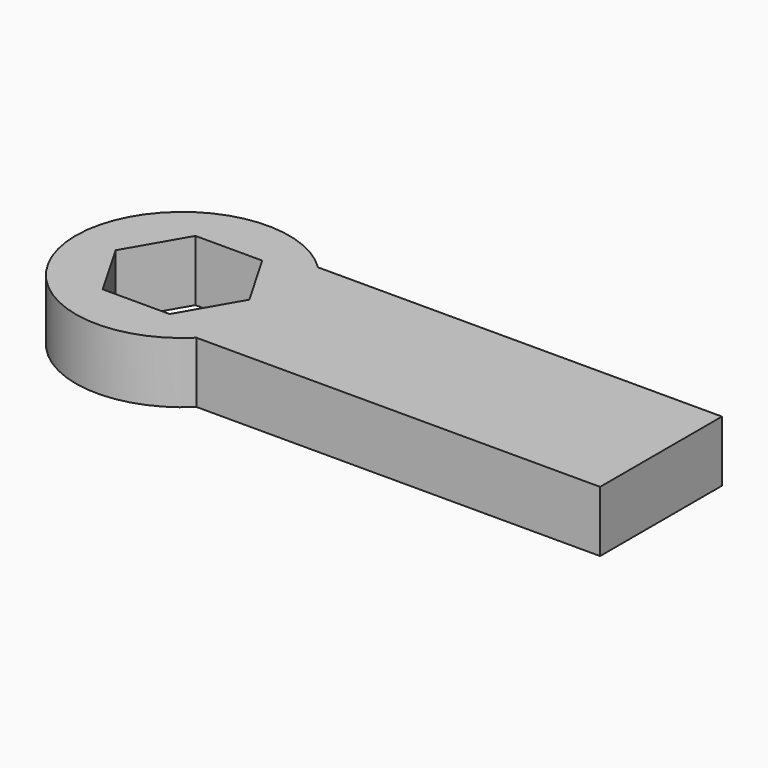
from build123d import *

# Parameters (mm, degrees)
F0_W     = 1257.3
F0_H     = 634.5049866525
F1_DEPTH = 254


# Not quite as in the source:
# - a feature names something its author has since deleted; it is built from what else it names


with BuildPart() as f1:
    # F0 (on Top) → F1 (new body)
    with BuildSketch(Plane.XY):
        with BuildLine():
            ThreePointArc((-425.0103845802, -317.0049866525), (-326.6720587383, -171.8701049425), (-292.1, 0))
            ThreePointArc((-292.1, 0), (-326.8088213402, 172.1959345996), (-425.5148026665, 317.5))
            ThreePointArc((-425.5148026665, 317.5), (-1181.09985954, -0.3533680164), (-425.0103845802, -317.0049866525))
        make_face()
        Polygon((-875.9146199555, 241.3), (-597.2853800445, 241.3), (-457.9707600891, 0), (-597.2853800445, -241.3), (-875.9146199555, -241.3), (-1015.2292399109, 0), align=None, mode=Mode.SUBTRACT)
        with Locations((628.65, 0.2475066738)):
            Rectangle(F0_W, F0_H)
        with BuildLine():
            ThreePointArc((-425.5148026665, 317.5), (-326.8088213402, 172.1959345996), (-292.1, 0))
            ThreePointArc((-292.1, 0), (-326.6720587383, -171.8701049425), (-425.0103845802, -317.0049866525))
            Line((-425.0103845802, -317.0049866525), (0, -317.0049866525))
            Line((0, -317.0049866525), (0, 317.5))
            Line((0, 317.5), (-425.5148026665, 317.5))
        make_face()
    extrude(amount=F1_DEPTH)


solid = f1.part
